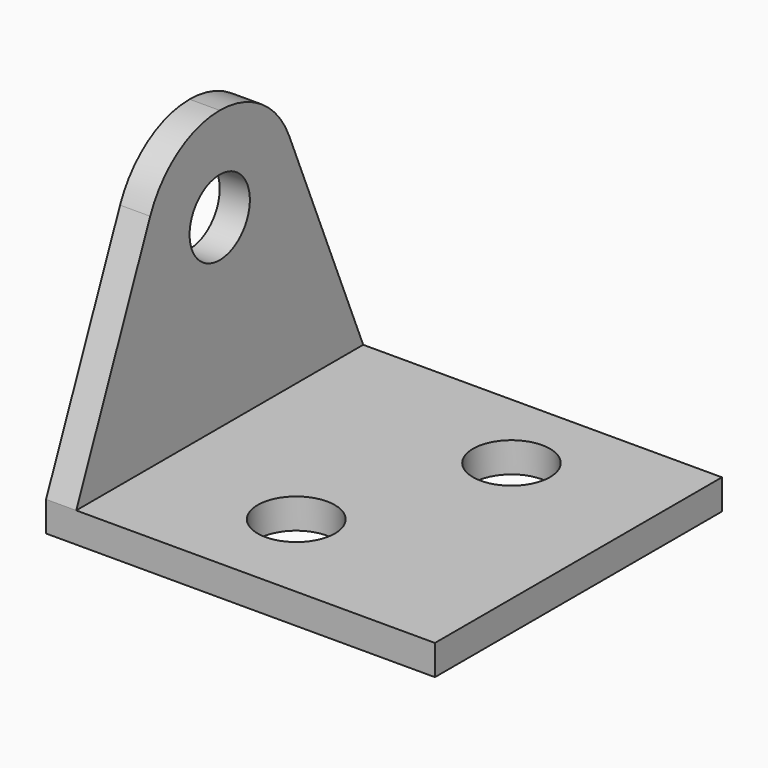
from build123d import *

# Parameters (mm, degrees)
F1_DEPTH = 9.525
F2_R     = 2
F3_DEPTH = 1.6002
F5_DEPTH = 1.6002
F6_R     = 2.0447
F6_R_2   = 2.05
F7_DEPTH = 1.6002


# Not quite as in the source:
# - a feature names something its author has since deleted; it is built from what else it names


with BuildPart() as f1:
    # F0 (on Front) → F1 (new body, symmetric)
    with BuildSketch(Plane.XZ):
        Polygon((1.6002, 19.05), (0, 19.05), (0, 0), (20.6502, 0), (20.6502, 1.6002), (1.6002, 1.6002), align=None)
    extrude(amount=F1_DEPTH, both=True)

    # F2 (on face) → F3 (cut, through all)
    with BuildSketch(Plane(origin=(0, 0, 0), x_dir=(0, -1, 0), z_dir=(-1, 0, 0))):
        with Locations((0, 11.43)):
            Circle(F2_R)
    extrude(amount=-F3_DEPTH, mode=Mode.SUBTRACT)

    # F4 (on face) → F5 (cut, through all)
    with BuildSketch(Plane(origin=(0, 0, 0), x_dir=(0, -1, 0), z_dir=(-1, 0, 0))):
        with BuildLine():
            Line((-9.525, 19.05), (-9.525, 1.6002))
            Line((-9.525, 1.6002), (-4.6136292969, 13.3572842838))
            ThreePointArc((-4.6136292969, 13.3572842838), (-2.7716041006, 15.5915154343), (0, 16.43))
            ThreePointArc((0, 16.43), (2.7716041006, 15.5915154343), (4.6136292969, 13.3572842838))
            Line((4.6136292969, 13.3572842838), (9.525, 1.6002))
            Line((9.525, 1.6002), (9.525, 19.05))
            Line((9.525, 19.05), (-9.525, 19.05))
        make_face()
    extrude(amount=-F5_DEPTH, mode=Mode.SUBTRACT)

    # F6 (on face) → F7 (cut, through all)
    with BuildSketch(Plane.XY.offset(1.6002)):
        with Locations((13.0302, 5.08)):
            Circle(F6_R)
        with Locations((9.2202, -4.445)):
            Circle(F6_R_2)
    extrude(amount=-F7_DEPTH, mode=Mode.SUBTRACT)


solid = f1.part
